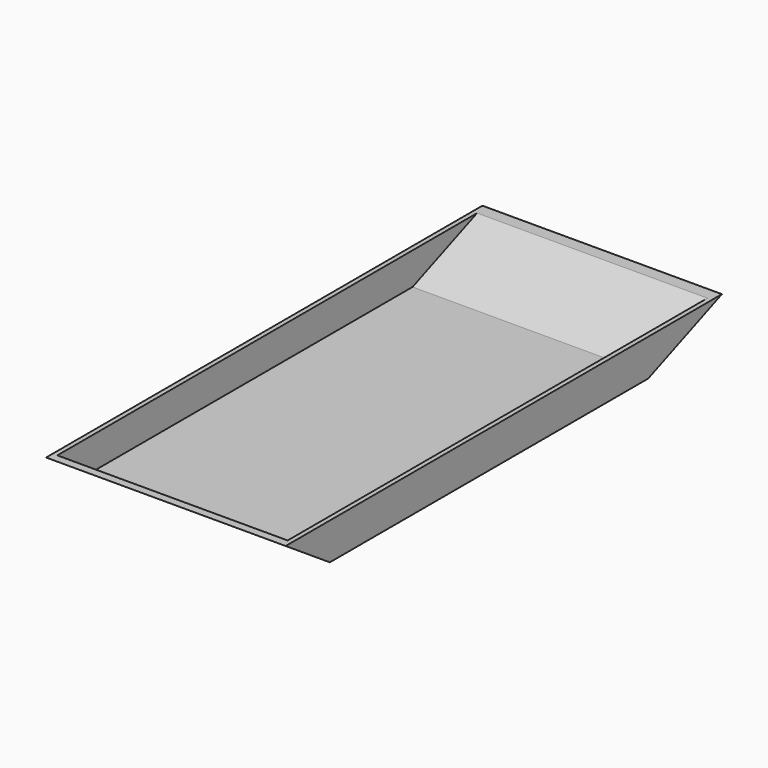
from build123d import *

# Parameters (mm, degrees)
F0_W     = 130
F0_H     = 296
F1_DEPTH = 10
F2_SIZE2 = 29.99999
F2_SIZE  = 19.99999
F3_SIZE2 = 19.99999
F3_SIZE  = 49.99999
F4_T     = 2.5


# Not quite as in the source:
# - a fillet or chamfer is up to 0.001 mm smaller than in the source, because OpenCascade refuses the exact size
# - a shell that OpenCascade refuses in one call is made with other operations: the cavity is built on its own and cut out


with BuildPart() as f1:
    # F0 (on Top) → F1 (new body, symmetric)
    with BuildSketch(Plane.XY):
        Rectangle(F0_W, F0_H)
    extrude(amount=F1_DEPTH, both=True)

    # F2 (size 20 and 30 in the source; OpenCascade refuses exactly that, so slightly less here)
    f2_edges = [f1.edges().sort_by_distance(p)[0] for p in [
        (0, -148, -10),
    ]]
    f2_side = f1.faces().sort_by_distance((0, -148, 0))[0]
    chamfer(f2_edges, length=F2_SIZE, length2=F2_SIZE2, reference=f2_side)

    # F3 (size 50 and 20 in the source; OpenCascade refuses exactly that, so slightly less here)
    f3_edges = [f1.edges().sort_by_distance(p)[0] for p in [
        (0, 148, -10),
    ]]
    f3_side = f1.faces().sort_by_distance((0, 14.999995, -10))[0]
    chamfer(f3_edges, length=F3_SIZE, length2=F3_SIZE2, reference=f3_side)

    # F4: shell of thickness 2.5, made by hand


with BuildPart() as f4_core1:
    # F4_t2: copy of F1
    add(f1.part)

    # the walls: a layer under each face that stays
    f4_faces = [f4_core1.faces().sort_by_distance(p)[0] for p in [
        (65, 0, 0),
        (0, -10, -10),
        (0, 123.000005, -5e-06),
        (0, -133.000005, -5e-06),
        (0, 148, 9.999995),
        (0, -148, 9.999995),
        (-65, 0, 0),
    ]]
    thicken(f4_faces, amount=-F4_T, mode=Mode.SUBTRACT)


with BuildPart() as f1_1:
    add(f1.part)

    # what is left inside the walls is the cavity
    f4_cavity = [f4_core1.part.solids().sort_by_distance(p)[0] for p in [
        (0, -48.572528, 9.975),
    ]]
    add(f4_cavity, mode=Mode.SUBTRACT)


solid = f1_1.part
